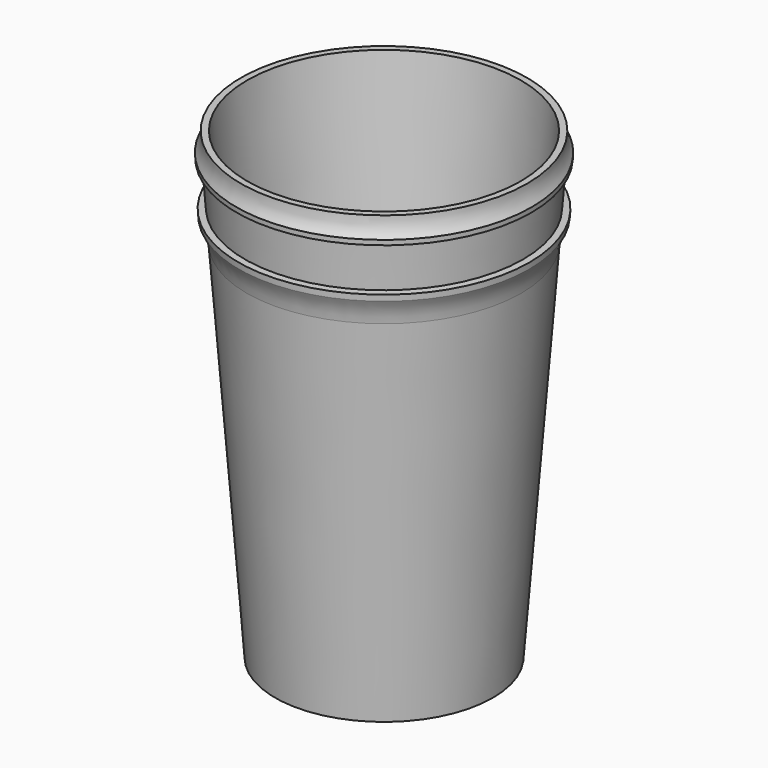
from build123d import *


# Not quite as in the source:
# - a fillet or chamfer that OpenCascade refuses, or shapes differently, is made with other operations: its cross-section is extruded or revolved along the edge and cut away or added


with BuildPart() as f2:
    # F0 (on Front) → F2 (revolve)
    with BuildSketch(Plane.XZ):
        Polygon((0, -52.5), (0, -57.5), (27, -57.5), (34.4796358746, 39.0916005051), (35.9751587861, 38.9757936776), (36.0909656136, 40.4713165891), (34.4796358746, 40.5960909966), (35.3289886101, 51.5645848486), (36.5399394434, 51.4708140523), (36.6354203483, 52.7038491323), (35.1398974369, 52.8196559599), (35.5, 57.4700003754), (33.9, 57.4700003754), (25.3843986885, -52.5), align=None)
    revolve(axis=Axis((0, 0, -0.416059047), (0, 0, -1)))

    # F3: fillet of radius 13 on 1 edges, made by hand

    # F3_s1 → F3_t2 (revolve)
    with BuildSketch(Plane.XZ):
        with BuildLine():
            ThreePointArc((34.0116081533, 33.0475166166), (34.6321139259, 36.1313140352), (35.9751587861, 38.9757936776))
            Line((35.9751587861, 38.9757936776), (34.4796358746, 39.0916005051))
            Line((34.4796358746, 39.0916005051), (34.0116081533, 33.0475166166))
        make_face()
    revolve(axis=Axis((0, 0, 39.0916005051), (0, 0, -1)))

    # F4: fillet of radius 8 on 1 edges, made by hand

    # F4_s1 → F4_t2 (revolve)
    with BuildSketch(Plane.XZ):
        with BuildLine():
            ThreePointArc((35.4999554959, 57.4694256524), (35.6939238208, 54.9975828995), (36.6354203483, 52.7038491323))
            Line((36.6354203483, 52.7038491323), (35.1398974369, 52.8196559599))
            Line((35.1398974369, 52.8196559599), (35.4999554959, 57.4694256524))
        make_face()
    revolve(axis=Axis((0, 0, 52.8196559599), (0, 0, -1)))


solid = f2.part
